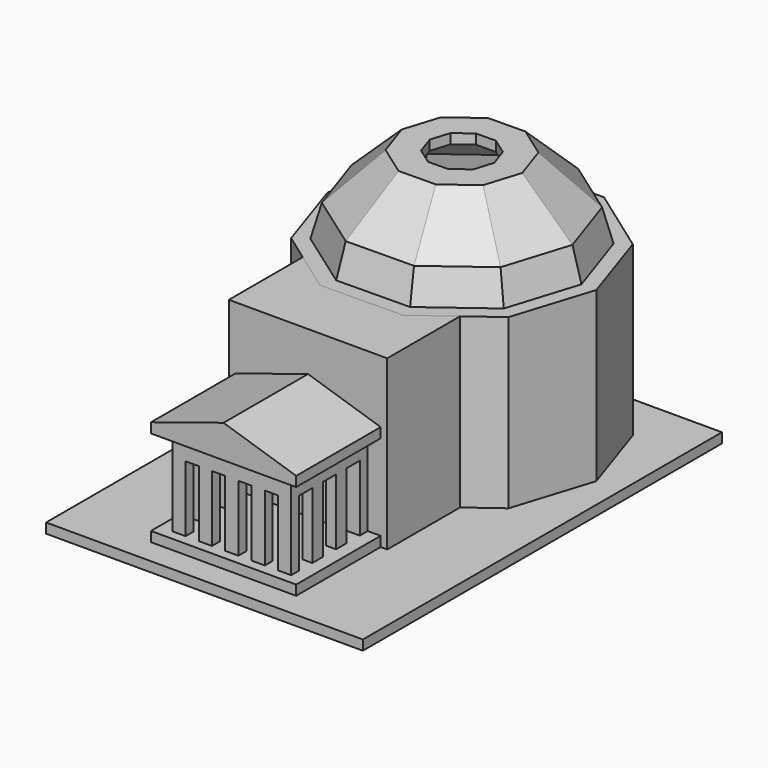
from build123d import *

# Parameters (mm, degrees)
F0_W      = 152.4
F0_H      = 215.9
F1_DEPTH  = 4.7625
F3_DEPTH  = 80.9625
F4_T      = -4.7625
F5_DEPTH  = 80.9635
F7_DEPTH  = 80.9625
F8_T      = -4.7625
F9_W      = 6.35
F9_H      = 4.7625
F9_W_2    = 4.7625
F9_H_2    = 6.35
F9_H_3    = 4.7752
F10_DEPTH = 4.7625
F11_W     = 6.35
F11_H     = 4.7752
F11_H_2   = 4.7625
F11_W_2   = 4.7625
F11_H_3   = 6.35
F12_DEPTH = 31.75
F15_W     = 57.15
F15_H     = 46.0375
F15_W_2   = 44.45
F15_H_2   = 36.5125
F16_DEPTH = 9.525
F17_W     = 69.85
F17_H     = 4.7625
F18_DEPTH = 50.8


# Not quite as in the source:
# - a feature names something its author has since deleted; it is built from what else it names


with BuildPart() as f1:
    # F0 (on Top) → F1 (new body)
    with BuildSketch(Plane.XY):
        with Locations((0.4908610135, 25.6078880154)):
            Rectangle(F0_W, F0_H)
    extrude(amount=F1_DEPTH)


with BuildPart() as f3:
    # F2 (on face) → F3 (new body)
    with BuildSketch(Plane.XY.offset(4.7625)):
        Polygon((19.8431090525, 133.7173784268), (-19.8431090525, 133.398397604), (-51.7624417186, 109.813362976), (-63.7227887654, 71.970956145), (-51.1557041384, 34.3256903041), (-18.8613870255, 11.2567774892), (20.8248310796, 11.5757583121), (52.7441637457, 35.16079294), (64.7045107925, 73.0031997711), (52.1374261654, 110.6484656119), align=None)
        Polygon((-36.3506679758, 98.6160539199), (-13.9563353097, 115.2807709686), (13.9563353097, 115.5997517914), (36.7256524226, 99.4511565558), (45.6545107925, 73.0031997711), (37.3323900028, 46.3581019962), (14.9380573368, 29.6933849475), (-12.9746132826, 29.3744041247), (-35.7439303955, 45.5229993603), (-44.6727887654, 71.970956145), align=None, mode=Mode.SUBTRACT)
        Polygon((13.9563353097, 115.5997517914), (-13.9563353097, 115.2807709686), (-36.3506679758, 98.6160539199), (-44.6727887654, 71.970956145), (-35.7439303955, 45.5229993603), (-12.9746132826, 29.3744041247), (14.9380573368, 29.6933849475), (37.3323900028, 46.3581019962), (45.6545107925, 73.0031997711), (36.7256524226, 99.4511565558), align=None)
    extrude(amount=F3_DEPTH)

    # F4
    f4_openings = [f3.faces().sort_by_distance(p)[0] for p in [
        (0.490861, 72.487078, 4.7625),
    ]]
    offset(amount=F4_T, openings=f4_openings)

    # F2 (on face) → F5 (cut, through all)
    with BuildSketch(Plane.XY.offset(4.7625)):
        Polygon((13.9563353097, 115.5997517914), (-13.9563353097, 115.2807709686), (-36.3506679758, 98.6160539199), (-44.6727887654, 71.970956145), (-35.7439303955, 45.5229993603), (-12.9746132826, 29.3744041247), (14.9380573368, 29.6933849475), (37.3323900028, 46.3581019962), (45.6545107925, 73.0031997711), (36.7256524226, 99.4511565558), align=None)
    extrude(amount=F5_DEPTH, mode=Mode.SUBTRACT)

    # F20: sweep along a path in F20_path
    with BuildLine(Plane(origin=(-35.7439303955, 45.5229993603, 85.725), x_dir=(0, -1, 0), z_dir=(0, 0, -1))) as f20_path:
        Line((0, 0), (16.1485952356, -22.7693171129))
        Line((16.1485952356, -22.7693171129), (15.8296144128, -50.6819877323))
        Line((15.8296144128, -50.6819877323), (-0.8351026359, -73.0763203984))
        Line((-0.8351026359, -73.0763203984), (-27.4802004108, -81.398441188))
        Line((-27.4802004108, -81.398441188), (-53.9281571955, -72.4695828181))
        Line((-53.9281571955, -72.4695828181), (-70.0767524311, -49.7002657052))
        Line((-70.0767524311, -49.7002657052), (-69.7577716083, -21.7875950858))
        Line((-69.7577716083, -21.7875950858), (-53.0930545596, 0.6067375802))
        Line((-53.0930545596, 0.6067375802), (-26.4479567847, 8.9288583699))
        Line((-26.4479567847, 8.9288583699), (0, 0))
    # F19 (on Right) → F20 (sweep)
    with BuildSketch(Plane.YZ):
        Polygon((22.392230299, 101.0590724923), (18.283477958, 85.725), (23.2139807672, 85.725), (26.6621709852, 98.5938210877), (47.1308498975, 119.0625), (57.8581578067, 119.0625), (57.8581578067, 123.825), (45.1581578067, 123.825), align=None)
    sweep(path=f20_path.line, transition=Transition.RIGHT)


with BuildPart() as f7:
    # F6 (on face) → F7 (new body)
    with BuildSketch(Plane.XY.offset(4.7625)):
        Polygon((-38.1, -19.4504366256), (38.1, -19.4504366256), (38.1, 24.3402938822), (20.8248310796, 11.5757583121), (-18.8613870255, 11.2567774892), (-38.1, 24.9995633744), align=None)
    extrude(amount=F7_DEPTH)

    # F8
    f8_openings = [f7.faces().sort_by_distance(p)[0] for p in [
        (-0.159074, -2.163387, 4.7625),
        (0.981722, 11.416268, 45.24375),
        (-28.480694, 18.12817, 45.24375),
        (29.462416, 17.958026, 45.24375),
    ]]
    offset(amount=F8_T, openings=f8_openings)


with BuildPart() as f10:
    # F9 (on face) → F10 (new body)
    with BuildSketch(Plane.XY.offset(4.7625)):
        Polygon((-34.925, -70.2504366256), (34.925, -70.2504366256), (34.925, -19.4504366256), (28.715682441, -19.4504366256), (28.715682441, -24.2129366256), (22.365682441, -24.2129366256), (22.365682441, -19.4504366256), (16.015682441, -19.4504366256), (16.015682441, -24.2256366256), (9.665682441, -24.2256366256), (9.665682441, -19.4504366256), (3.315682441, -19.4504366256), (3.315682441, -24.2256366256), (-3.034317559, -24.2256366256), (-3.034317559, -19.4504366256), (-9.384317559, -19.4504366256), (-9.384317559, -24.2256366256), (-15.734317559, -24.2256366256), (-15.734317559, -19.4504366256), (-22.084317559, -19.4504366256), (-22.084317559, -24.2256366256), (-28.434317559, -24.2256366256), (-28.434317559, -19.4504366256), (-34.925, -19.4504366256), align=None)
        with Locations((-25.259317559, -63.1066866256)):
            Rectangle(F9_W, F9_H, mode=Mode.SUBTRACT)
        with Locations((-12.559317559, -63.1066866256)):
            Rectangle(F9_W, F9_H, mode=Mode.SUBTRACT)
        with Locations((0.140682441, -63.1066866256)):
            Rectangle(F9_W, F9_H, mode=Mode.SUBTRACT)
        with Locations((-26.053067559, -49.6129366256)):
            Rectangle(F9_W_2, F9_H_2, mode=Mode.SUBTRACT)
        with Locations((-26.053067559, -35.3254366256)):
            Rectangle(F9_W_2, F9_H_2, mode=Mode.SUBTRACT)
        with Locations((12.840682441, -63.1066866256)):
            Rectangle(F9_W, F9_H, mode=Mode.SUBTRACT)
        with Locations((25.540682441, -63.1066866256)):
            Rectangle(F9_W, F9_H, mode=Mode.SUBTRACT)
        with Locations((26.334432441, -49.6129366256)):
            Rectangle(F9_W_2, F9_H_2, mode=Mode.SUBTRACT)
        with Locations((26.334432441, -35.3254366256)):
            Rectangle(F9_W_2, F9_H_2, mode=Mode.SUBTRACT)
        with Locations((12.840682441, -21.8380366256)):
            Rectangle(F9_W, F9_H_3)
        with Locations((0.140682441, -21.8380366256)):
            Rectangle(F9_W, F9_H_3)
        with Locations((-12.559317559, -21.8380366256)):
            Rectangle(F9_W, F9_H_3)
        with Locations((-25.259317559, -21.8380366256)):
            Rectangle(F9_W, F9_H_3)
        with Locations((25.540682441, -21.8316866256)):
            Rectangle(F9_W, F9_H)
        with Locations((-26.053067559, -49.6129366256)):
            Rectangle(F9_W_2, F9_H_2)
        with Locations((-25.259317559, -63.1066866256)):
            Rectangle(F9_W, F9_H)
        with Locations((-26.053067559, -35.3254366256)):
            Rectangle(F9_W_2, F9_H_2)
        with Locations((-12.559317559, -63.1066866256)):
            Rectangle(F9_W, F9_H)
        with Locations((26.334432441, -35.3254366256)):
            Rectangle(F9_W_2, F9_H_2)
        with Locations((26.334432441, -49.6129366256)):
            Rectangle(F9_W_2, F9_H_2)
        with Locations((25.540682441, -63.1066866256)):
            Rectangle(F9_W, F9_H)
        with Locations((12.840682441, -63.1066866256)):
            Rectangle(F9_W, F9_H)
        with Locations((0.140682441, -63.1066866256)):
            Rectangle(F9_W, F9_H)
    extrude(amount=F10_DEPTH)

    # F11 (on face) → F12 (join)
    with BuildSketch(Plane.XY.offset(9.525)):
        with Locations((-25.259317559, -21.8380366256)):
            Rectangle(F11_W, F11_H)
        with Locations((25.540682441, -21.8316866256)):
            Rectangle(F11_W, F11_H_2)
        with Locations((12.840682441, -21.8380366256)):
            Rectangle(F11_W, F11_H)
        with Locations((0.140682441, -21.8380366256)):
            Rectangle(F11_W, F11_H)
        with Locations((-12.559317559, -21.8380366256)):
            Rectangle(F11_W, F11_H)
        with Locations((-26.053067559, -35.3254366256)):
            Rectangle(F11_W_2, F11_H_3)
        with Locations((-26.053067559, -49.6129366256)):
            Rectangle(F11_W_2, F11_H_3)
        with Locations((-25.259317559, -63.1066866256)):
            Rectangle(F11_W, F11_H_2)
        with Locations((-12.559317559, -63.1066866256)):
            Rectangle(F11_W, F11_H_2)
        with Locations((0.140682441, -63.1066866256)):
            Rectangle(F11_W, F11_H_2)
        with Locations((12.840682441, -63.1066866256)):
            Rectangle(F11_W, F11_H_2)
        with Locations((25.540682441, -63.1066866256)):
            Rectangle(F11_W, F11_H_2)
        with Locations((26.334432441, -49.6129366256)):
            Rectangle(F11_W_2, F11_H_3)
        with Locations((26.334432441, -35.3254366256)):
            Rectangle(F11_W_2, F11_H_3)
    extrude(amount=F12_DEPTH)

    # F15 (on face) → F16 (join)
    with BuildSketch(Plane.XY.offset(41.275)):
        with Locations((0.140682441, -42.4691866256)):
            Rectangle(F15_W, F15_H)
        with Locations((0.140682441, -42.4691866256)):
            Rectangle(F15_W_2, F15_H_2, mode=Mode.SUBTRACT)
    extrude(amount=F16_DEPTH)

    # F17 (on face) → F18 (join)
    with BuildSketch(Plane.XZ.offset(19.4504366256)):
        with Locations((0, 53.18125)):
            Rectangle(F17_W, F17_H)
        Polygon((0, 66.675), (-34.925, 55.5625), (34.925, 55.5625), align=None)
    extrude(amount=F18_DEPTH)


solid = Compound([f1.part, f3.part, f7.part, f10.part])
